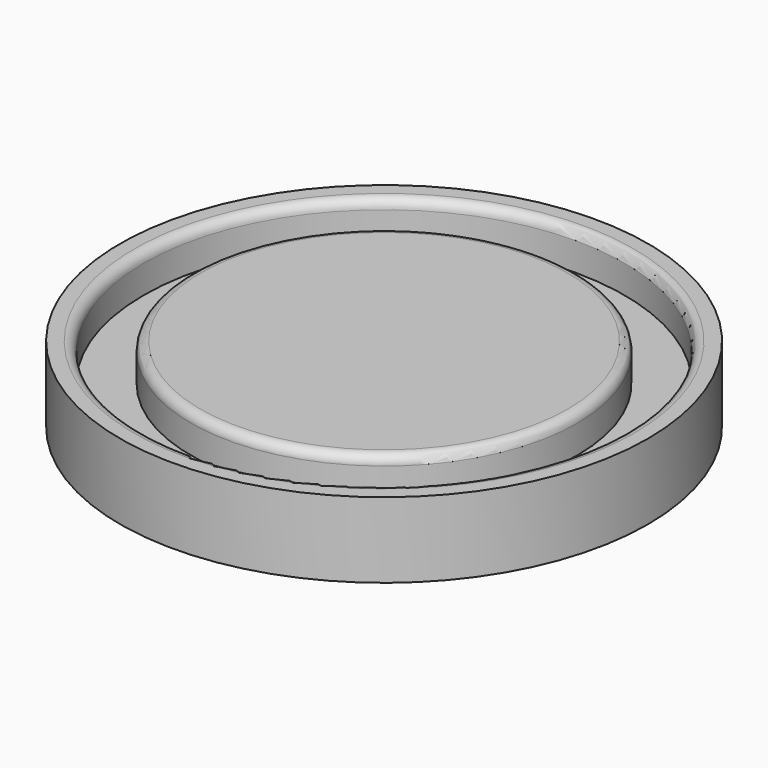
from build123d import *

# Parameters (mm, degrees)
F0_R     = 14
F0_R_2   = 12.75
F0_R_3   = 10.25
F1_DEPTH = 2
F2_DEPTH = 4
F3_R     = 0.5
F4_R     = 0.5


with BuildPart() as f1:
    # F0 (on Top) → F1 (new body)
    with BuildSketch(Plane.XY):
        Circle(F0_R)
        Circle(F0_R_2, mode=Mode.SUBTRACT)
        Circle(F0_R_2)
        Circle(F0_R_3, mode=Mode.SUBTRACT)
        Circle(F0_R_3)
    extrude(amount=F1_DEPTH)


with BuildPart() as f2:
    # F0 (on Top) → F2 (new body)
    with BuildSketch(Plane.XY):
        Circle(F0_R)
        Circle(F0_R_2, mode=Mode.SUBTRACT)
    extrude(amount=F2_DEPTH)

    # F4
    f4_edges = [f2.edges().sort_by_distance(p)[0] for p in [
        (-12.75, 0, 4),
    ]]
    fillet(f4_edges, radius=F4_R)


with BuildPart() as f2b:
    # F0 (on Top) → F2, piece 2 (new body)
    with BuildSketch(Plane.XY):
        Circle(F0_R_3)
    extrude(amount=F2_DEPTH)

    # F3
    f3_edges = [f2b.edges().sort_by_distance(p)[0] for p in [
        (-10.25, 0, 4),
    ]]
    fillet(f3_edges, radius=F3_R)


solid = Compound([f1.part, f2.part, f2b.part])
